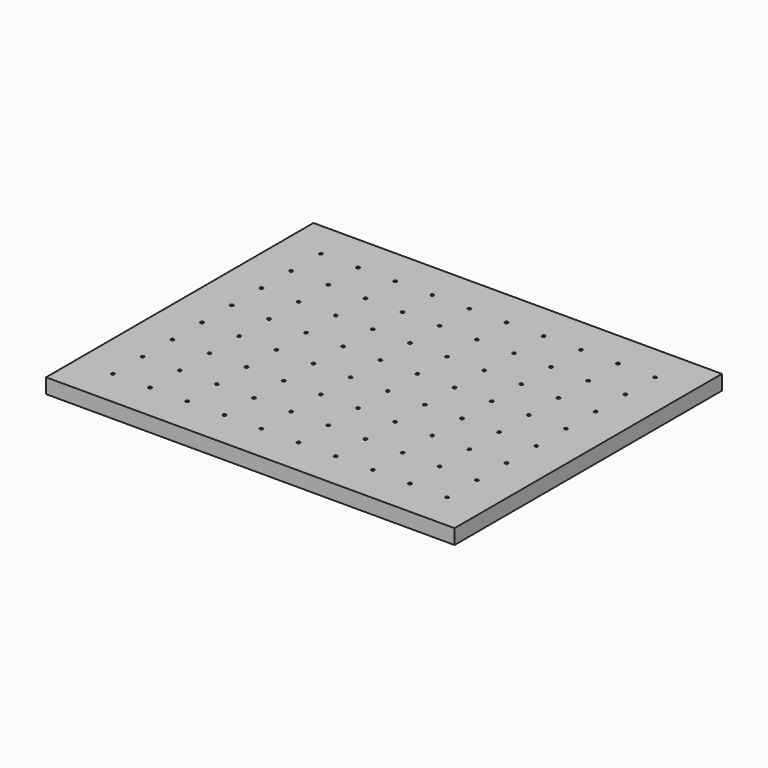
from build123d import *

# Parameters (mm, degrees)
F0_W     = 1100
F0_H     = 900
F1_DEPTH = 40
F3_D     = 8.4328


with BuildPart() as f1:
    # F0 (on Top) → F1 (new body)
    with BuildSketch(Plane.XY):
        Rectangle(F0_W, F0_H)
    extrude(amount=F1_DEPTH)

    # F3 (through all)
    with Locations(Plane.XY.offset(40)):
        with Locations((-450, -350), (-350, -350), (-250, -350), (-450, -250), (-350, -250), (-250, -250), (-150, -150), (-50, -250), (-150, -350), (-250, -150), (-150, -250), (350, -50), (-450, 150), (-450, -50), (-450, 50), (-450, 250), (-450, 350), (450, 50), (250, 50), (50, 50), (-150, 50), (150, 350), (-50, 350), (-250, 350), (350, 350), (150, 150), (-50, 150), (-250, 150), (350, 150), (150, -50), (-50, -50), (-250, -50), (450, -150), (350, -250), (250, -150), (150, -250), (50, -150), (-350, 350), (450, 350), (250, 350), (50, 350), (-150, 350), (-350, 150), (450, 150), (250, 150), (50, 150), (-150, 150), (250, -350), (50, -350), (450, -350), (150, 250), (-50, 250), (-250, 250), (350, 250), (150, 50), (-50, 50), (-250, 50), (350, 50), (450, -50), (250, -50), (350, -150), (50, -50), (150, -150), (-150, -50), (-50, -150), (450, -250), (250, -250), (350, -350), (50, -250), (150, -350), (-50, -350), (-350, 250), (-350, -150), (-350, -50), (450, 250), (250, 250), (50, 250), (-150, 250), (-350, 50), (-450, -150)):
            Hole(F3_D / 2)


solid = f1.part
